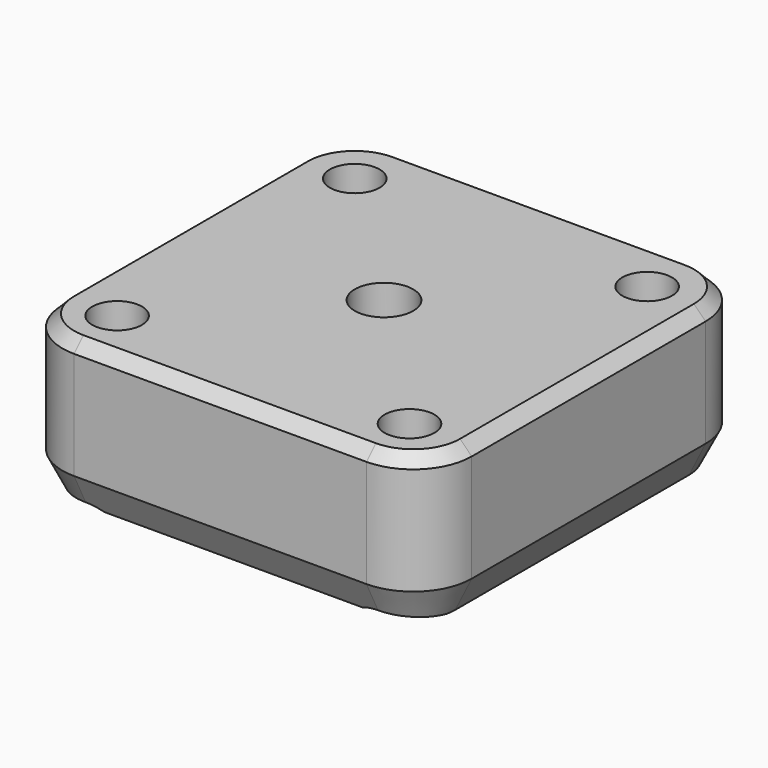
from build123d import *

# Parameters (mm, degrees)
F0_W         = 35
F0_H         = 35
F1_DEPTH     = 6.5
F2_R         = 2.125
F3_DEPTH     = 13.001
F4_R         = 5
F5_T1_DEPTH  = 25
F5_T3_DEPTH  = 25
F5_T12_ANGLE = 90
F5_T14_ANGLE = 90
F5_T16_ANGLE = 90
F5_T18_ANGLE = 90
F6_R         = 2.5
F7_DEPTH     = 13.001
F8_SIZE      = 1


# Not quite as in the source:
# - a fillet or chamfer that OpenCascade refuses, or shapes differently, is made with other operations: its cross-section is extruded or revolved along the edge and cut away or added


with BuildPart() as f1:
    # F0 (on Top) → F1 (new body, symmetric)
    with BuildSketch(Plane.XY):
        Rectangle(F0_W, F0_H)
    extrude(amount=F1_DEPTH, both=True)

    # F2 (on face) → F3 (cut, through all)
    with BuildSketch(Plane.XY.offset(6.5)):
        with Locations((-12.5, -12.9)):
            Circle(F2_R)
        with Locations((-12.5, 12.5)):
            Circle(F2_R)
        with Locations((12.5, 12.5)):
            Circle(F2_R)
        with Locations((12.5, -12.9)):
            Circle(F2_R)
    extrude(amount=-F3_DEPTH, mode=Mode.SUBTRACT)

    # F4
    f4_edges = [f1.edges().sort_by_distance(p)[0] for p in [
        (-17.5, 17.5, 0),
        (17.5, 17.5, 0),
        (17.5, -17.5, 0),
        (-17.5, -17.5, 0),
    ]]
    fillet(f4_edges, radius=F4_R)

    # F5: chamfer of 1.4 x 2.8 on 12 edges, made by hand

    # F5_s2 → F5_t1 (cut)
    with BuildSketch(Plane.XZ.offset(-12.5)):
        Polygon((17.5, -3.7), (16.1, -6.5), (17.5, -6.5), align=None)
        Polygon((-16.1, -6.5), (-17.5, -3.7), (-17.5, -6.5), align=None)
    extrude(amount=F5_T1_DEPTH, mode=Mode.SUBTRACT)

    # F5_s4 → F5_t3 (cut)
    with BuildSketch(Plane.YZ.offset(-12.5)):
        Polygon((-16.1, -6.5), (-17.5, -3.7), (-17.5, -6.5), align=None)
        Polygon((16.1, -6.5), (17.5, -3.7), (17.5, -6.5), align=None)
    extrude(amount=F5_T3_DEPTH, mode=Mode.SUBTRACT)

    # F5_s5 → F5_t6 (revolve, cut)
    with BuildSketch(Plane.XZ.offset(12.9)):
        Polygon((-8.975, -6.5), (-10.375, -3.7), (-10.375, -6.5), align=None)
    revolve(axis=Axis((-12.5, -12.9, -6.5), (0, 0, 1)), mode=Mode.SUBTRACT)

    # F5_s7 → F5_t8 (revolve, cut)
    with BuildSketch(Plane.XZ.offset(12.9)):
        Polygon((16.025, -6.5), (14.625, -3.7), (14.625, -6.5), align=None)
    revolve(axis=Axis((12.5, -12.9, -6.5), (0, 0, 1)), mode=Mode.SUBTRACT)

    # F5_s9 → F5_t10 (revolve, cut)
    with BuildSketch(Plane.XZ.offset(-12.5)):
        Polygon((16.025, -6.5), (14.625, -3.7), (14.625, -6.5), align=None)
    revolve(axis=Axis((12.5, 12.5, -6.5), (0, 0, 1)), mode=Mode.SUBTRACT)

    # F5_s11 → F5_t12 (revolve, cut)
    with BuildSketch(Plane.XZ.offset(12.5)):
        Polygon((16.1, -6.5), (17.5, -3.7), (17.5, -6.5), align=None)
    revolve(axis=Axis((12.5, -12.5, -6.5), (0, 0, -1)), revolution_arc=F5_T12_ANGLE, mode=Mode.SUBTRACT)

    # F5_s13 → F5_t14 (revolve, cut)
    with BuildSketch(Plane.XZ.offset(-12.5)):
        Polygon((16.1, -6.5), (17.5, -3.7), (17.5, -6.5), align=None)
    revolve(axis=Axis((12.5, 12.5, -6.5), (0, 0, 1)), revolution_arc=F5_T14_ANGLE, mode=Mode.SUBTRACT)

    # F5_s15 → F5_t16 (revolve, cut)
    with BuildSketch(Plane.YZ.offset(-12.5)):
        Polygon((-16.1, -6.5), (-17.5, -3.7), (-17.5, -6.5), align=None)
    revolve(axis=Axis((-12.5, -12.5, -6.5), (0, 0, -1)), revolution_arc=F5_T16_ANGLE, mode=Mode.SUBTRACT)

    # F5_s17 → F5_t18 (revolve, cut)
    with BuildSketch(Plane.YZ.offset(-12.5)):
        Polygon((16.1, -6.5), (17.5, -3.7), (17.5, -6.5), align=None)
    revolve(axis=Axis((-12.5, 12.5, -6.5), (0, 0, 1)), revolution_arc=F5_T18_ANGLE, mode=Mode.SUBTRACT)

    # F5_s19 → F5_t20 (revolve, cut)
    with BuildSketch(Plane.XZ.offset(-12.5)):
        Polygon((-8.975, -6.5), (-10.375, -3.7), (-10.375, -6.5), align=None)
    revolve(axis=Axis((-12.5, 12.5, -6.5), (0, 0, 1)), mode=Mode.SUBTRACT)

    # F6 (on face) → F7 (cut, through all)
    with BuildSketch(Plane(origin=(0, 0, -6.5), x_dir=(1, 0, 0), z_dir=(0, 0, -1))):
        Circle(F6_R)
    extrude(amount=-F7_DEPTH, mode=Mode.SUBTRACT)

    # F8
    f8_edges = [f1.edges().sort_by_distance(p)[0] for p in [
        (-17.5, 0, 6.5),
    ]]
    chamfer(f8_edges, length=F8_SIZE)


solid = f1.part
